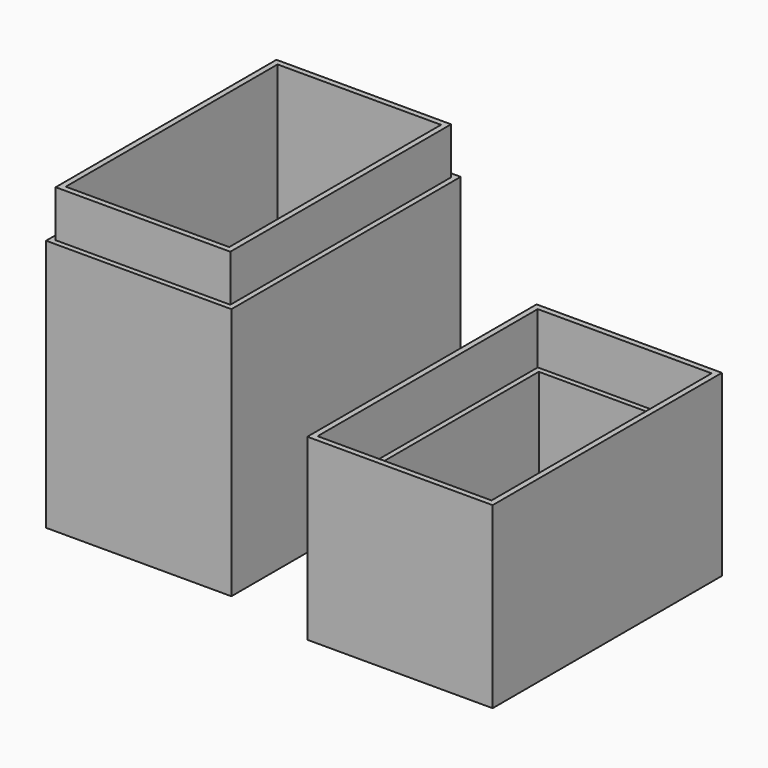
from build123d import *

# Parameters (mm, degrees)
F0_W          = 39.7
F0_H          = 61.4
F1_DEPTH      = 54.15
F2_W          = 37.42
F2_H          = 59.12
F3_DEPTH      = 10
F4_W          = 35.02
F4_H          = 56.72
F5_DEPTH      = 62.1
F6_W          = 39.7
F6_H          = 61.4
F7_DEPTH      = 38.3
F8_W          = 37.26
F8_H          = 58.96
F9_DEPTH      = 11
F10_W         = 35.02
F10_H         = 56.72
F11_DEPTH     = 25.4
F12_W         = 35.3
F12_H         = 56.05
F13_DEPTH     = 87.1
F15_TEXT_SIZE = 22.3545216715
F16_DEPTH     = 1


# Not quite as in the source:
# - Text() gives the source's letters only with a copy of the font that has no kerning and outlines rounded to 1/6400 em; it was checked with that copy


with BuildPart() as f1:
    # F0 (on Top) → F1 (new body)
    with BuildSketch(Plane.XY):
        with Locations((-33.0157025415, 4.0777856603)):
            Rectangle(F0_W, F0_H)
    extrude(amount=F1_DEPTH)

    # F2 (on face) → F3 (join)
    with BuildSketch(Plane.XY.offset(54.15)):
        with Locations((-33.0157025415, 4.0777856603)):
            Rectangle(F2_W, F2_H)
    extrude(amount=F3_DEPTH)

    # F4 (on face) → F5 (cut)
    with BuildSketch(Plane.XY.offset(64.15)):
        with Locations((-33.0157025415, 4.0777856603)):
            Rectangle(F4_W, F4_H)
    extrude(amount=-F5_DEPTH, mode=Mode.SUBTRACT)

    # F15 (on face) → F16 (join)
    with BuildSketch(Plane(origin=(-52.8657025415, 0, 0), x_dir=(0, -1, 0), z_dir=(-1, 0, 0))):
        with Locations((-28.7777856603, 28.6429295738)):
            Text('UNO', F15_TEXT_SIZE, font='Open Sans', font_style=FontStyle.BOLDITALIC, text_align=(TextAlign.LEFT, TextAlign.BOTTOM))
    extrude(amount=F16_DEPTH)


with BuildPart() as f7:
    # F6 (on Top) → F7 (new body)
    with BuildSketch(Plane.XY):
        with Locations((26.4462144114, -0.2911494041)):
            Rectangle(F6_W, F6_H)
    extrude(amount=F7_DEPTH)

    # F8 (on face) → F9 (cut)
    with BuildSketch(Plane.XY.offset(38.3)):
        with Locations((26.4462144114, -0.2911494041)):
            Rectangle(F8_W, F8_H)
    extrude(amount=-F9_DEPTH, mode=Mode.SUBTRACT)

    # F10 (on face) → F11 (cut)
    with BuildSketch(Plane.XY.offset(27.3)):
        with Locations((26.4462144114, -0.2911494041)):
            Rectangle(F10_W, F10_H)
    extrude(amount=-F11_DEPTH, mode=Mode.SUBTRACT)


with BuildPart() as f13:
    # F12 (on Top) → F13 (new body)
    with BuildSketch(Plane.XY):
        with Locations((-22.3607545537, 67.1475064522)):
            Rectangle(F12_W, F12_H)
    extrude(amount=F13_DEPTH)


solid = Compound([f1.part, f7.part])
